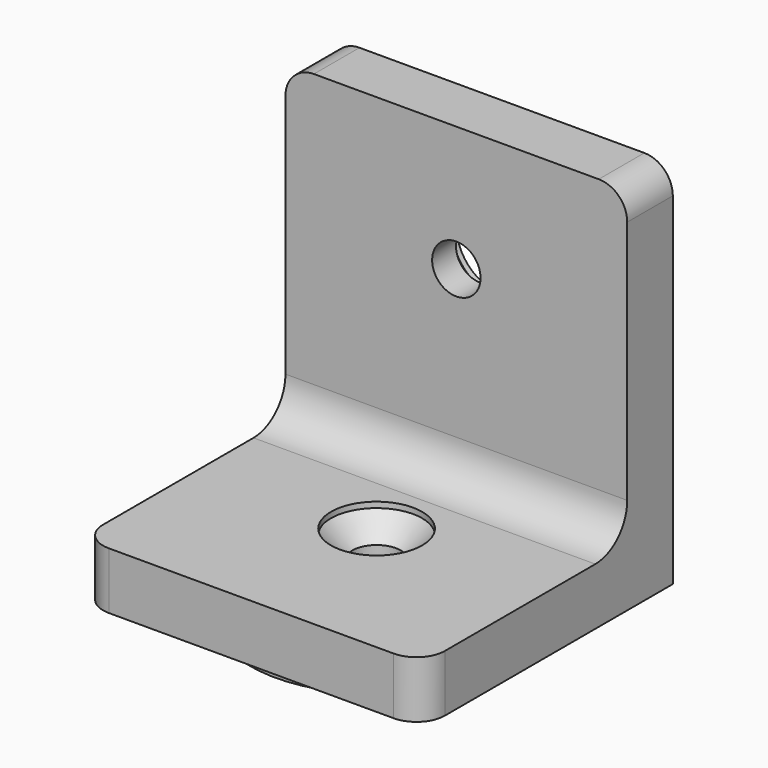
from build123d import *

# Parameters (mm, degrees)
F1_DEPTH  = 60
F2_R      = 22.25
F3_DEPTH  = 4
F4_R      = 4.25
F5_DEPTH  = 25
F6_R      = 8
F7_DEPTH  = 1
F8_SIZE   = 3.74999
F9_R      = 4.25
F10_DEPTH = 25
F11_R     = 8
F12_DEPTH = 1
F13_SIZE  = 3.74999
F14_R     = 5
F15_R     = 7


# Not quite as in the source:
# - a fillet or chamfer is up to 0.001 mm smaller than in the source, because OpenCascade refuses the exact size


with BuildPart() as f1:
    # F0 (on Right) → F1 (new body)
    with BuildSketch(Plane.YZ):
        Polygon((32.3616418088, -17.0859274204), (32.3616418088, 47.9140725796), (22.3616418088, 47.9140725796), (22.3616418088, -7.0859274204), (-22.6383581912, -7.0859274204), (-22.6383581912, -17.0859274204), align=None)
    extrude(amount=F1_DEPTH)

    # F2 (on face) → F3 (join)
    with BuildSketch(Plane(origin=(0, 0, -17.0859274204), x_dir=(1, 0, 0), z_dir=(0, 0, -1))):
        with Locations((30, -4.8616418088)):
            Circle(F2_R)
    extrude(amount=F3_DEPTH)

    # F4 (on face) → F5 (cut)
    with BuildSketch(Plane(origin=(0, 0, -21.0859274204), x_dir=(1, 0, 0), z_dir=(0, 0, -1))):
        with Locations((30, -4.8616418088)):
            Circle(F4_R)
    extrude(amount=-F5_DEPTH, mode=Mode.SUBTRACT)

    # F6 (on face) → F7 (cut)
    with BuildSketch(Plane.XY.offset(-7.0859274204)):
        with Locations((30, 4.8616418088)):
            Circle(F6_R)
    extrude(amount=-F7_DEPTH, mode=Mode.SUBTRACT)

    # F8 (size 3.75 in the source; OpenCascade refuses exactly that, so slightly less here)
    f8_edges = [f1.edges().sort_by_distance(p)[0] for p in [
        (25.75, 4.861642, -8.085927),
    ]]
    chamfer(f8_edges, length=F8_SIZE)

    # F9 (on face) → F10 (cut)
    with BuildSketch(Plane(origin=(0, 32.3616418088, 0), x_dir=(-1, 0, 0), z_dir=(0, 1, 0))):
        with Locations((-30, 25.9140725796)):
            Circle(F9_R)
    extrude(amount=-F10_DEPTH, mode=Mode.SUBTRACT)

    # F11 (on face) → F12 (cut)
    with BuildSketch(Plane(origin=(0, 32.3616418088, 0), x_dir=(-1, 0, 0), z_dir=(0, 1, 0))):
        with Locations((-30, 25.9140725796)):
            Circle(F11_R)
    extrude(amount=-F12_DEPTH, mode=Mode.SUBTRACT)

    # F13 (size 3.75 in the source; OpenCascade refuses exactly that, so slightly less here)
    f13_edges = [f1.edges().sort_by_distance(p)[0] for p in [
        (34.25, 31.361642, 25.914073),
    ]]
    chamfer(f13_edges, length=F13_SIZE)

    # F14
    f14_edges = [f1.edges().sort_by_distance(p)[0] for p in [
        (0, -22.638358, -12.085927),
        (60, -22.638358, -12.085927),
        (60, 27.361642, 47.914073),
        (0, 27.361642, 47.914073),
    ]]
    fillet(f14_edges, radius=F14_R)

    # F15
    f15_edges = [f1.edges().sort_by_distance(p)[0] for p in [
        (30, 22.361642, -7.085927),
    ]]
    fillet(f15_edges, radius=F15_R)


solid = f1.part
